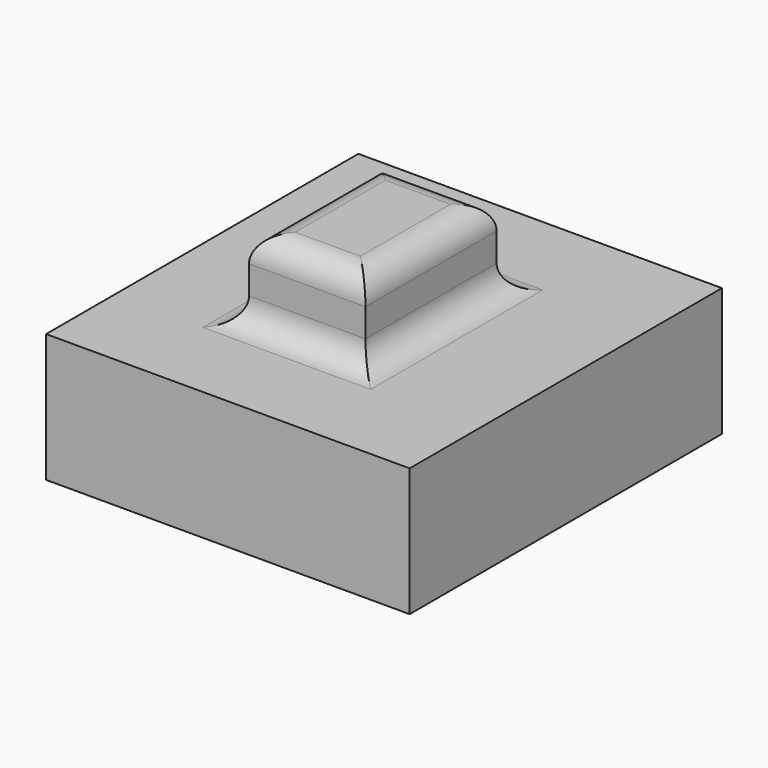
from build123d import *

# Parameters (mm, degrees)
F0_W     = 23.0411533266
F0_H     = 32.4329454452
F1_DEPTH = 41.148
F2_W     = 71.9308368862
F2_H     = 77.2322397679
F3_DEPTH = 25.4
F4_R     = 5.08
F5_W     = 45.4457737505
F5_H     = 51.1372797191
F6_DEPTH = 7.62
F7_R     = 0.5842
F8_DEPTH = 7.62


with BuildPart() as f1:
    # F0 (on Top) → F1 (new body)
    with BuildSketch(Plane.XY):
        with Locations((-11.5205766633, -9.9749034271)):
            Rectangle(F0_W, F0_H)
    extrude(amount=F1_DEPTH)

    # F2 (on Top) → F3 (join)
    with BuildSketch(Plane.XY):
        with Locations((-9.6630994231, -9.5305936411)):
            Rectangle(F2_W, F2_H)
    extrude(amount=F3_DEPTH)

    # F4
    f4_edges = [f1.edges().sort_by_distance(p)[0] for p in [
        (-23.041153, -9.974903, 25.4),
        (-11.520577, -26.191376, 25.4),
        (0, -9.974903, 25.4),
        (-11.520577, 6.241569, 25.4),
        (-11.520577, 6.241569, 41.148),
        (-23.041153, -9.974903, 41.148),
        (-11.520577, -26.191376, 41.148),
        (0, -9.974903, 41.148),
    ]]
    fillet(f4_edges, radius=F4_R)


with BuildPart() as f6:
    # F5 (on Top) → F6 (new body)
    with BuildSketch(Plane.XY):
        Rectangle(F5_W, F5_H)
    extrude(amount=F6_DEPTH)

    # F7 (on face) → F8 (cut, through all)
    with BuildSketch(Plane.XY.offset(7.62)):
        with Locations((10.16, -10.16)):
            Circle(F7_R)
        with Locations((10.16, 10.16)):
            Circle(F7_R)
        with Locations((-10.16, 10.16)):
            Circle(F7_R)
        with Locations((-10.16, -10.16)):
            Circle(F7_R)
    extrude(amount=-F8_DEPTH, mode=Mode.SUBTRACT)


solid = Compound([f1.part, f6.part])
